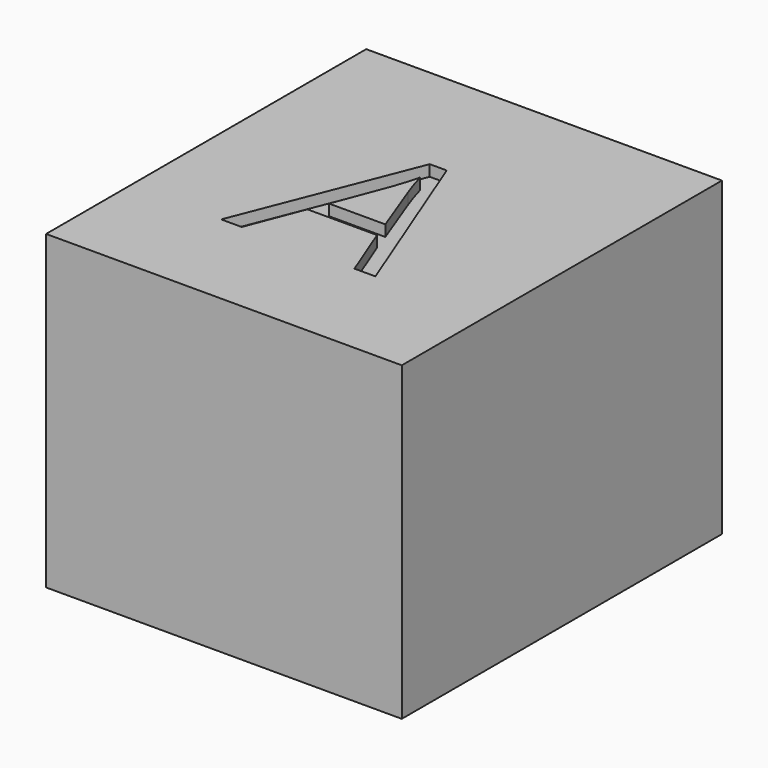
from build123d import *

# Parameters (mm, degrees)
F0_W         = 812.8
F0_H         = 711.2
F1_DEPTH     = 457.2
F2_TEXT_SIZE = 556.8500815166
F3_DEPTH     = 25.4


# Not quite as in the source:
# - Text() gives the source's letters only with a copy of the font that has no kerning and outlines rounded to 1/6400 em; it was checked with that copy


with BuildPart() as f1:
    # F0 (on Front) → F1 (new body, symmetric)
    with BuildSketch(Plane.XZ):
        Rectangle(F0_W, F0_H)
    extrude(amount=F1_DEPTH, both=True)

    # F2 (on face) → F3 (cut)
    with BuildSketch(Plane.XY.offset(355.6)):
        with Locations((-197.4223703146, -218.2481437922)):
            Text('A', F2_TEXT_SIZE, font='Open Sans', text_align=(TextAlign.LEFT, TextAlign.BOTTOM))
    extrude(amount=-F3_DEPTH, mode=Mode.SUBTRACT)


solid = f1.part
